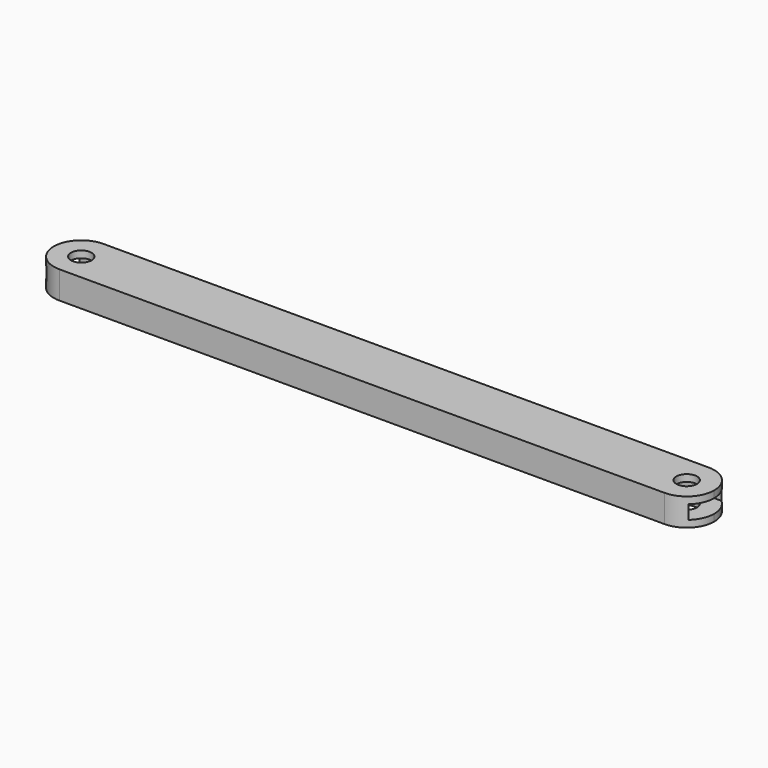
from build123d import *

# Parameters (mm, degrees)
F0_W          = 304.8
F0_H          = 25.4
F1_DEPTH      = 6.35
F2_R          = 12.69999
F3_R          = 4.7625
F4_DEPTH      = 12.701
F5_W          = 19.05
F5_H          = 6.35
F6_DEPTH      = 152.401
F6_DEPTH_BACK = 152.401


# Not quite as in the source:
# - a fillet or chamfer is up to 0.001 mm smaller than in the source, because OpenCascade refuses the exact size


with BuildPart() as f1:
    # F0 (on Top) → F1 (new body, symmetric)
    with BuildSketch(Plane.XY):
        Rectangle(F0_W, F0_H)
    extrude(amount=F1_DEPTH, both=True)

    # F2 (radius 12.7 in the source; OpenCascade refuses exactly that, so slightly less here)
    f2_edges = [f1.edges().sort_by_distance(p)[0] for p in [
        (-152.4, 12.7, 0),
        (-152.4, -12.7, 0),
        (152.4, 12.7, 0),
        (152.4, -12.7, 0),
    ]]
    fillet(f2_edges, radius=F2_R)

    # F3 (on face) → F4 (cut, through all)
    with BuildSketch(Plane.XY.offset(6.35)):
        with Locations((-139.7, 0)):
            Circle(F3_R)
        with Locations((139.7, 0)):
            Circle(F3_R)
    extrude(amount=-F4_DEPTH, mode=Mode.SUBTRACT)

    # F5 (on Right) → F6 (cut, two sides)
    with BuildSketch(Plane.YZ) as f6_sk:
        Rectangle(F5_W, F5_H)
    extrude(amount=-F6_DEPTH, mode=Mode.SUBTRACT)
    extrude(f6_sk.sketch, amount=F6_DEPTH_BACK, mode=Mode.SUBTRACT)


solid = f1.part
